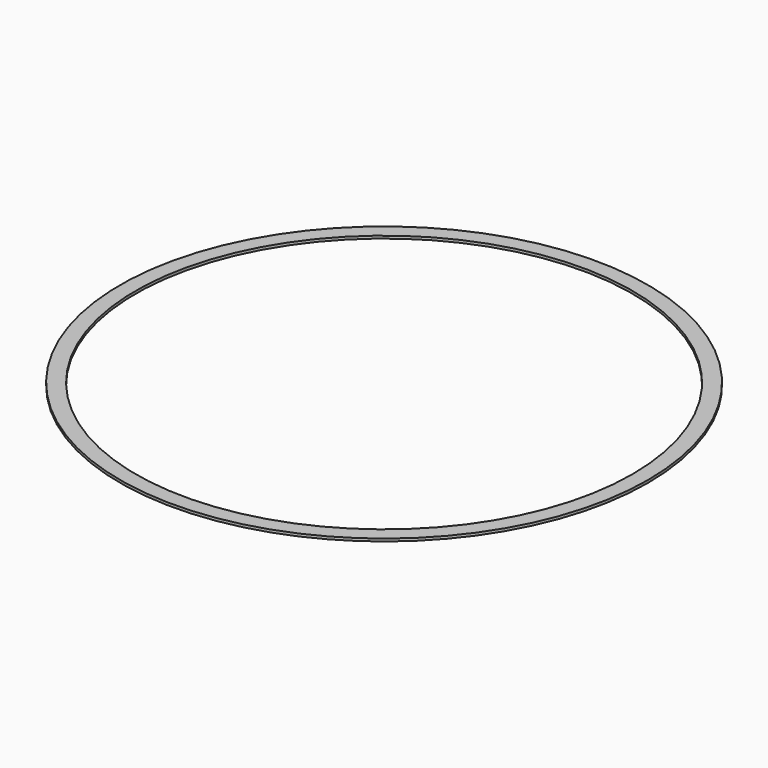
from build123d import *

# Parameters (mm, degrees)
F0_R     = 429.89246
F0_R_2   = 404.49246
F1_DEPTH = 4.2333333333


# Not quite as in the source:
# - a length typed as a fraction of an inch, garbled in the dataset ("3 / 203.2 mm" for 3/8 in), is restored


with BuildPart() as f1:
    # F0 (on Top) → F1 (new body)
    with BuildSketch(Plane.XY):
        Circle(F0_R)
        Circle(F0_R_2, mode=Mode.SUBTRACT)
    extrude(amount=F1_DEPTH)


solid = f1.part
